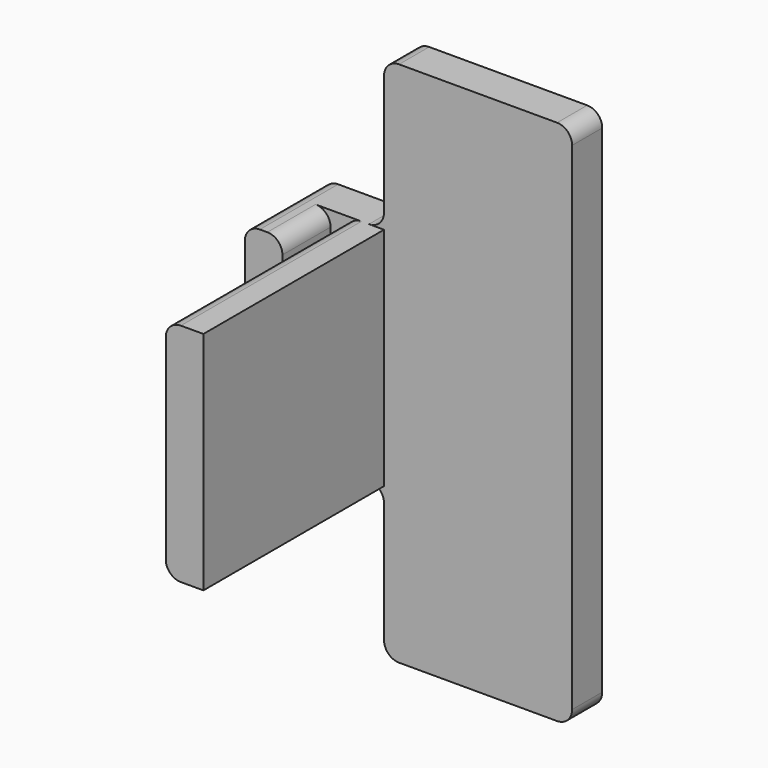
from build123d import *

# Parameters (mm, degrees)
F1_DEPTH = 15
F0_W     = 25
F0_H     = 5
F2_DEPTH = 35
F3_R     = 2


with BuildPart() as f1:
    # F0 (on Top) → F1 (new body, symmetric)
    with BuildSketch(Plane.XY):
        Polygon((-12.1, 0), (-12.1, -13), (-7.1, -13), (-7.1, -5), (-5, -5), (-5, -35), (0, -35), (0, -5), (0, 0), align=None)
    extrude(amount=F1_DEPTH, both=True)

    # F0 (on Top) → F2 (join, symmetric)
    with BuildSketch(Plane.XY):
        with Locations((12.5, -2.5)):
            Rectangle(F0_W, F0_H)
    extrude(amount=F2_DEPTH, both=True)

    # F3
    f3_edges = [f1.edges().sort_by_distance(p)[0] for p in [
        (0, -2.5, 15),
        (0, -2.5, -15),
        (0, -2.5, -35),
        (0, -2.5, 35),
        (25, -2.5, 35),
        (25, -2.5, -35),
        (-12.1, -6.5, 15),
        (-5, -20, 15),
        (-7.1, -9, 15),
        (-5, -20, -15),
        (-12.1, -6.5, -15),
        (-7.1, -9, -15),
    ]]
    fillet(f3_edges, radius=F3_R)


solid = f1.part
